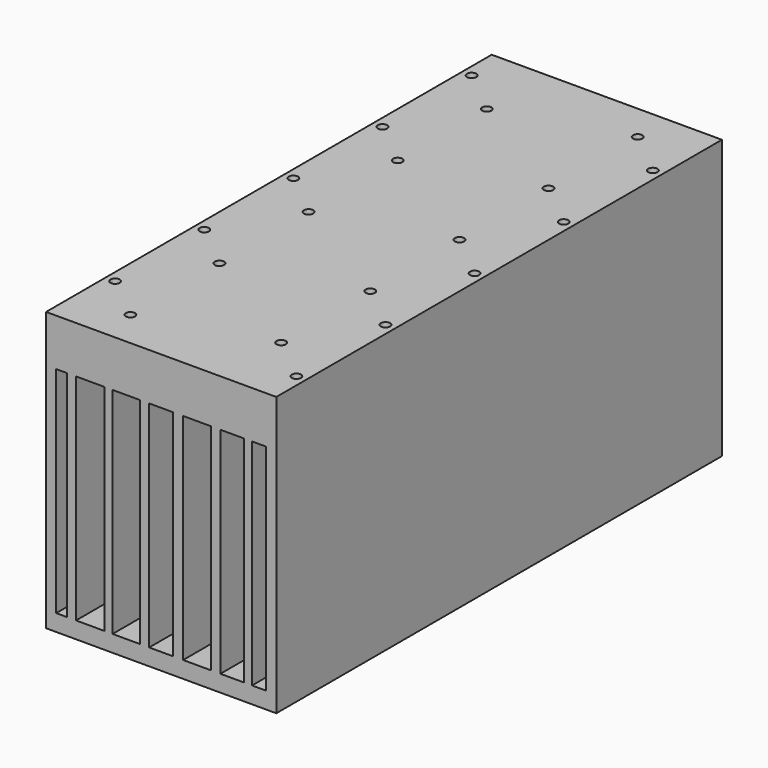
from build123d import *

# Parameters (mm, degrees)
F0_W     = 62
F0_H     = 150
F0_R     = 1.25
F1_DEPTH = 12
F2_W     = 62
F2_H     = 150
F3_DEPTH = 63
F4_W     = 3.7979930639
F4_H     = 57.8553974628
F4_W_2   = 6.3762590289
F4_W_3   = 7.4440259486
F4_W_4   = 6.4508207142
F4_W_5   = 7.4439314194
F4_W_6   = 7.6164929196
F4_W_7   = 2.9675979167
F5_DEPTH = 150


# Not quite as in the source:
# - a feature names something its author has since deleted; it is built from what else it names


with BuildPart() as f1:
    # F0 (on Top) → F1 (new body)
    with BuildSketch(Plane.XY):
        Rectangle(F0_W, F0_H)
        with Locations((-16.35, -64.95)):
            Circle(F0_R, mode=Mode.SUBTRACT)
        with Locations((-28.4, -55)):
            Circle(F0_R, mode=Mode.SUBTRACT)
        with Locations((-28.4, -25)):
            Circle(F0_R, mode=Mode.SUBTRACT)
        with Locations((-16.35, -34.95)):
            Circle(F0_R, mode=Mode.SUBTRACT)
        with Locations((-16.35, -4.95)):
            Circle(F0_R, mode=Mode.SUBTRACT)
        with Locations((28.4, -65)):
            Circle(F0_R, mode=Mode.SUBTRACT)
        with Locations((16.35, -55.05)):
            Circle(F0_R, mode=Mode.SUBTRACT)
        with Locations((16.35, -25.05)):
            Circle(F0_R, mode=Mode.SUBTRACT)
        with Locations((28.4, -35)):
            Circle(F0_R, mode=Mode.SUBTRACT)
        with Locations((28.4, -5)):
            Circle(F0_R, mode=Mode.SUBTRACT)
        with Locations((-28.4, 5)):
            Circle(F0_R, mode=Mode.SUBTRACT)
        with Locations((-28.4, 35)):
            Circle(F0_R, mode=Mode.SUBTRACT)
        with Locations((-16.35, 25.05)):
            Circle(F0_R, mode=Mode.SUBTRACT)
        with Locations((-16.35, 55.05)):
            Circle(F0_R, mode=Mode.SUBTRACT)
        with Locations((-28.4, 65)):
            Circle(F0_R, mode=Mode.SUBTRACT)
        with Locations((16.35, 4.95)):
            Circle(F0_R, mode=Mode.SUBTRACT)
        with Locations((16.35, 34.95)):
            Circle(F0_R, mode=Mode.SUBTRACT)
        with Locations((28.4, 25)):
            Circle(F0_R, mode=Mode.SUBTRACT)
        with Locations((28.4, 55)):
            Circle(F0_R, mode=Mode.SUBTRACT)
        with Locations((16.35, 64.95)):
            Circle(F0_R, mode=Mode.SUBTRACT)
    extrude(amount=-F1_DEPTH)

    # F2 (on face) → F3 (join)
    with BuildSketch(Plane(origin=(0, 0, -12), x_dir=(1, 0, 0), z_dir=(0, 0, -1))):
        Rectangle(F2_W, F2_H)
    extrude(amount=F3_DEPTH)

    # F4 (on face) → F5 (cut)
    with BuildSketch(Plane(origin=(0, 75, 0), x_dir=(-1, 0, 0), z_dir=(0, 1, 0))):
        with Locations((-26.3689886779, -41.5959060192)):
            Rectangle(F4_W, F4_H)
        with Locations((-19.1375147551, -41.5959060192)):
            Rectangle(F4_W_2, F4_H)
        with Locations((-9.6363741904, -41.5959060192)):
            Rectangle(F4_W_3, F4_H)
        with Locations((0, -41.5959060192)):
            Rectangle(F4_W_4, F4_H)
        with Locations((9.3659532722, -41.5959060192)):
            Rectangle(F4_W_5, F4_H)
        with Locations((19.1261232831, -41.5959060192)):
            Rectangle(F4_W_6, F4_H)
        with Locations((26.7841862515, -41.5959060192)):
            Rectangle(F4_W_7, F4_H)
    extrude(amount=-F5_DEPTH, mode=Mode.SUBTRACT)


solid = f1.part
